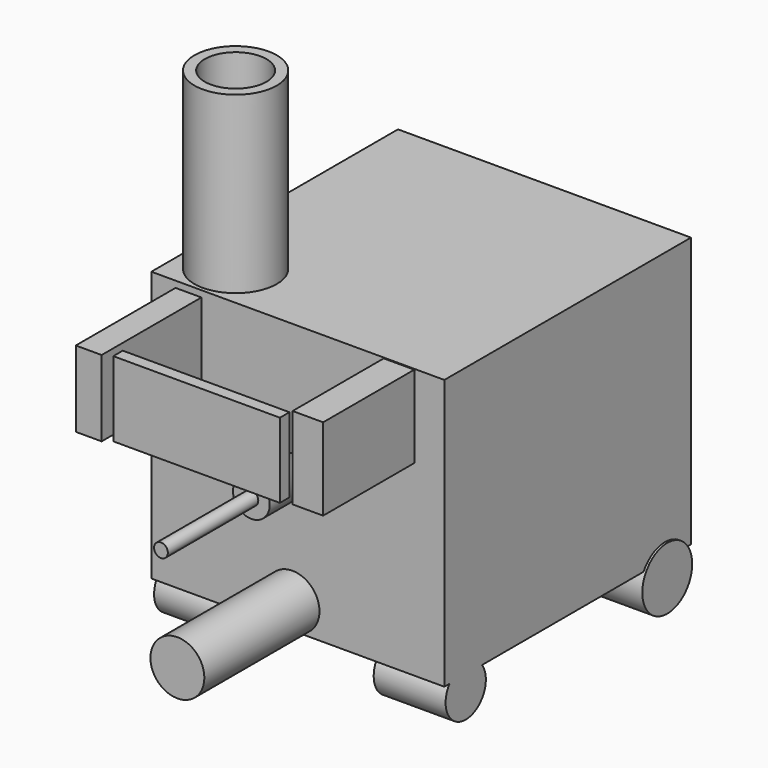
from build123d import *

# Parameters (mm, degrees)
F0_W      = 72.4286958575
F0_H      = 66.7624995112
F1_DEPTH  = 76.2
F2_R      = 10.1703504115
F3_DEPTH  = 43.18
F4_R      = 6.6667791351
F5_DEPTH  = 35.56
F6_R      = 7.7108976591
F7_DEPTH  = 38.1
F8_R      = 7.9071951907
F9_DEPTH  = 35.56
F11_DEPTH = 17.78
F14_R     = 4.5374330057
F15_DEPTH = 12.7
F20_W     = 6.3906405121
F20_H     = 30.8254435658
F21_DEPTH = 18.796
F22_W     = 7.5489785522
F22_H     = 28.1635001302
F23_DEPTH = 20.32
F24_W     = 41.1858335137
F24_H     = 2.9357820749
F25_DEPTH = 18.542
F27_D     = 15.24
F28_R     = 6.0147196054
F29_DEPTH = 16.256
F30_R     = 1.7038843718
F31_DEPTH = 27.94


with BuildPart() as f1:
    # F0 (on Front) → F1 (new body)
    with BuildSketch(Plane.XZ):
        with Locations((1.3298764825, -0.6317384541)):
            Rectangle(F0_W, F0_H)
    extrude(amount=F1_DEPTH)

    # F2 (on face) → F3 (join)
    with BuildSketch(Plane.XY.offset(32.7495113015)):
        with Locations((-22.9268483818, -65.106138587)):
            Circle(F2_R)
    extrude(amount=F3_DEPTH)

    # F4 (on face) → F5 (join)
    with BuildSketch(Plane.XZ.offset(76.2)):
        with Locations((0, -27.6431385428)):
            Circle(F4_R)
    extrude(amount=F5_DEPTH)

    # F6 (on Right) → F7 (join)
    with BuildSketch(Plane.YZ):
        with Locations((-8.026397787, -37.9476025701)):
            Circle(F6_R)
    extrude(amount=F7_DEPTH)

    # F8 (on face) → F9 (join)
    with BuildSketch(Plane(origin=(0, 0, 0), x_dir=(0, -1, 0), z_dir=(-1, 0, 0))):
        with Locations((8.026397787, -37.9476025701)):
            Circle(F8_R)
    extrude(amount=F9_DEPTH)

    # F10 (on face) → F11 (join)
    with BuildSketch(Plane.YZ.offset(37.5442244112)):
        with BuildLine():
            ThreePointArc((-74.6429898938, -34.0129882097), (-71.5028168985, -43.5598665716), (-63.3792777676, -37.6427993178))
            ThreePointArc((-63.3792777676, -37.6427993178), (-63.678932762, -35.735982435), (-64.5490101377, -34.0129882097))
            Line((-64.5490101377, -34.0129882097), (-74.6429898938, -34.0129882097))
        make_face()
    extrude(amount=-F11_DEPTH)

    # F14 (on face) → F15 (join)
    with BuildSketch(Plane.XZ.offset(76.2)):
        Circle(F14_R)
    extrude(amount=F15_DEPTH)

    # F27 (through all)
    with Locations(Plane.XY.offset(75.9295113015)):
        with Locations((-22.9268483818, -65.106138587)):
            Hole(F27_D / 2)

    # F28 (on face) → F29 (join)
    with BuildSketch(Plane(origin=(-34.8844714463, 0, 0), x_dir=(0, -1, 0), z_dir=(-1, 0, 0))):
        with Locations((69.3431347609, -37.7799607813)):
            Circle(F28_R)
    extrude(amount=-F29_DEPTH)

    # F30 (on face) → F31 (join)
    with BuildSketch(Plane.XZ.offset(88.9)):
        Circle(F30_R)
    extrude(amount=F31_DEPTH)


with BuildPart() as f21:
    # F20 (on face) → F21 (new body)
    with BuildSketch(Plane(origin=(0, 0, 12.6491999254), x_dir=(1, 0, 0), z_dir=(0, 0, -1))):
        with Locations((-25.3745997325, 92.0241959393)):
            Rectangle(F20_W, F20_H)
    extrude(amount=-F21_DEPTH)


with BuildPart() as f23:
    # F22 (on face) → F23 (new body)
    with BuildSketch(Plane(origin=(0, 0, 12.6491999254), x_dir=(1, 0, 0), z_dir=(0, 0, -1))):
        with Locations((26.8225362524, 90.8939503133)):
            Rectangle(F22_W, F22_H)
    extrude(amount=-F23_DEPTH)


with BuildPart() as f25:
    # F24 (on face) → F25 (new body)
    with BuildSketch(Plane(origin=(0, 0, 12.6491999254), x_dir=(1, 0, 0), z_dir=(0, 0, -1))):
        with Locations((0.1522358507, 104.5498177409)):
            Rectangle(F24_W, F24_H)
    extrude(amount=-F25_DEPTH)


solid = Compound([f1.part, f21.part, f23.part, f25.part])
